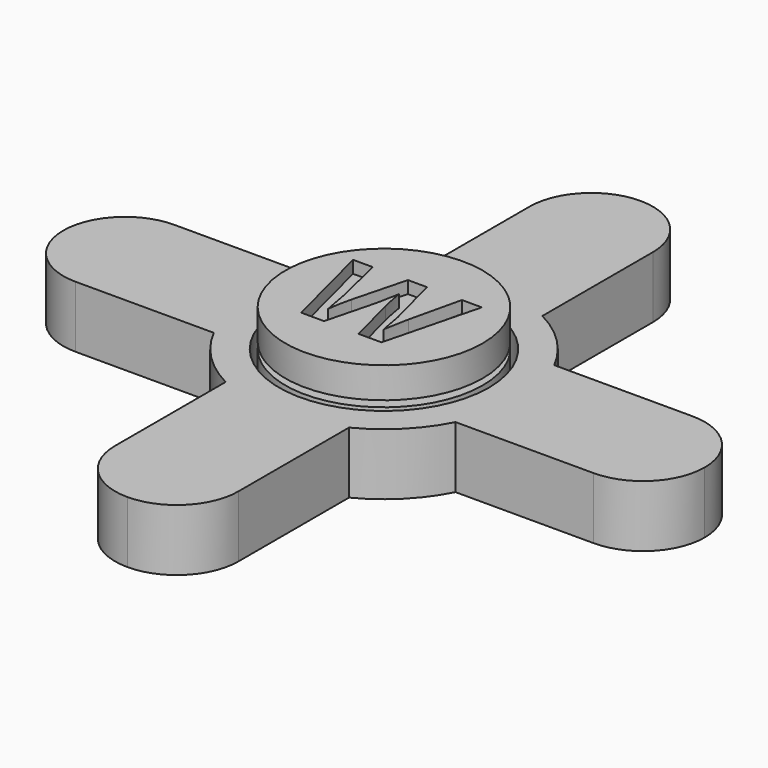
from build123d import *

# Parameters (mm, degrees)
F0_R         = 16
F0_R_2       = 6.5
F1_DEPTH     = 10
F0_R_3       = 17
F3_R         = 6
F4_DEPTH     = 6
F5_R         = 16
F5_R_2       = 6
F6_DEPTH     = 5
F7_TEXT_SIZE = 21.6005647938
F8_DEPTH     = 2
F9_R         = 9.99999
F10_R        = 8.5
F10_R_2      = 6
F11_DEPTH    = 1


# Not quite as in the source:
# - a fillet or chamfer is up to 0.001 mm smaller than in the source, because OpenCascade refuses the exact size
# - a feature names something its author has since deleted; it is built from what else it names
# - Text() gives the source's letters only with a copy of the font that has no kerning and outlines rounded to 1/6400 em; it was checked with that copy


with BuildPart() as f1:
    # F0 (on Top) → F1 (new body)
    with BuildSketch(Plane.XY):
        Circle(F0_R)
        Circle(F0_R_2, mode=Mode.SUBTRACT)
    extrude(amount=F1_DEPTH)


with BuildPart() as f1b:
    # F0 (on Top) → F1, piece 2 (new body)
    with BuildSketch(Plane.XY):
        with BuildLine():
            ThreePointArc((19.5959179423, -10), (21.3905375661, -5.1424607568), (22, 0))
            ThreePointArc((22, 0), (21.3905375661, 5.1424607568), (19.5959179423, 10))
            ThreePointArc((19.5959179423, 10), (15.5563491861, 15.5563491861), (10, 19.5959179423))
            ThreePointArc((10, 19.5959179423), (0, 22), (-10, 19.5959179423))
            ThreePointArc((-10, 19.5959179423), (-15.5563491861, 15.5563491861), (-19.5959179423, 10))
            ThreePointArc((-19.5959179423, 10), (-22, 0), (-19.5959179423, -10))
            ThreePointArc((-19.5959179423, -10), (-15.5563491861, -15.5563491861), (-10, -19.5959179423))
            ThreePointArc((-10, -19.5959179423), (0, -22), (10, -19.5959179423))
            ThreePointArc((10, -19.5959179423), (15.5563491861, -15.5563491861), (19.5959179423, -10))
        make_face()
        Circle(F0_R_3, mode=Mode.SUBTRACT)
        with BuildLine():
            ThreePointArc((19.5959179423, 10), (21.3905375661, 5.1424607568), (22, 0))
            ThreePointArc((22, 0), (21.3905375661, -5.1424607568), (19.5959179423, -10))
            Line((19.5959179423, -10), (52, -10))
            Line((52, -10), (52, 10))
            Line((52, 10), (19.5959179423, 10))
        make_face()
        with BuildLine():
            ThreePointArc((-10, 19.5959179423), (0, 22), (10, 19.5959179423))
            Line((10, 19.5959179423), (10, 52))
            Line((10, 52), (-10, 52))
            Line((-10, 52), (-10, 19.5959179423))
        make_face()
        with BuildLine():
            Line((10, -52), (10, -19.5959179423))
            ThreePointArc((10, -19.5959179423), (0, -22), (-10, -19.5959179423))
            Line((-10, -19.5959179423), (-10, -52))
            Line((-10, -52), (10, -52))
        make_face()
        with BuildLine():
            ThreePointArc((-19.5959179423, -10), (-22, 0), (-19.5959179423, 10))
            Line((-19.5959179423, 10), (-52, 10))
            Line((-52, 10), (-52, -10))
            Line((-52, -10), (-19.5959179423, -10))
        make_face()
    extrude(amount=F1_DEPTH)

    # F9 (radius 10 in the source; OpenCascade refuses exactly that, so slightly less here)
    f9_edges = [f1b.edges().sort_by_distance(p)[0] for p in [
        (-52, -10, 5),
        (-52, 10, 5),
        (-10, 52, 5),
        (10, 52, 5),
        (52, 10, 5),
        (52, -10, 5),
        (10, -52, 5),
        (-10, -52, 5),
    ]]
    fillet(f9_edges, radius=F9_R)


with BuildPart() as f4:
    # F3 (on offset) → F4 (new body)
    with BuildSketch(Plane.XY.offset(5)):
        Circle(F3_R)
    extrude(amount=F4_DEPTH)


with BuildPart() as f6:
    # F5 (on face) → F6 (new body)
    with BuildSketch(Plane.XY.offset(11)):
        Circle(F5_R)
        Circle(F5_R_2, mode=Mode.SUBTRACT)
        Circle(F5_R_2)
    extrude(amount=F6_DEPTH)

    # F7 (on face) → F8 (cut)
    with BuildSketch(Plane.XY.offset(16)):
        with Locations((-11.1428538542, -7.7762033258)):
            Text('W', F7_TEXT_SIZE, font='Open Sans', font_style=FontStyle.BOLD, text_align=(TextAlign.LEFT, TextAlign.BOTTOM))
    extrude(amount=-F8_DEPTH, mode=Mode.SUBTRACT)


with BuildPart() as f11:
    # F10 (on face) → F11 (new body)
    with BuildSketch(Plane(origin=(0, 0, 11), x_dir=(1, 0, 0), z_dir=(0, 0, -1))):
        Circle(F10_R)
        Circle(F10_R_2, mode=Mode.SUBTRACT)
    extrude(amount=F11_DEPTH)


solid = Compound([f1.part, f1b.part, f4.part, f6.part, f11.part])
